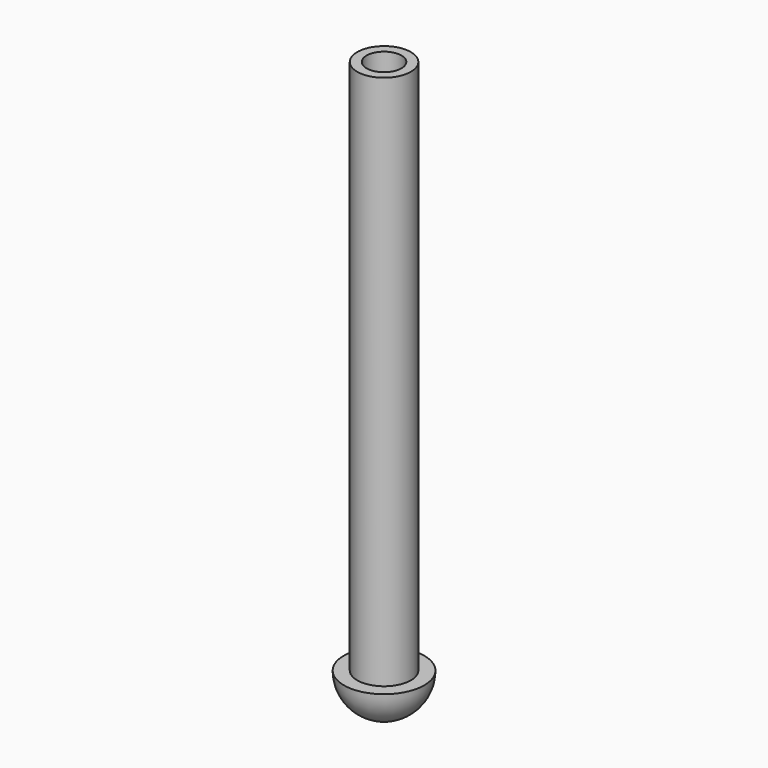
from build123d import *

# Parameters (mm, degrees)
F0_R     = 2.54
F1_DEPTH = 50.8
F3_R     = 1.651
F4_DEPTH = 6.35
F5_R     = 3.81
F6_DEPTH = 3.81
F7_R     = 3.80999


# Not quite as in the source:
# - a fillet or chamfer is up to 0.001 mm smaller than in the source, because OpenCascade refuses the exact size


with BuildPart() as f1:
    # F0 (on Top) → F1 (new body)
    with BuildSketch(Plane.XY):
        Circle(F0_R)
    extrude(amount=F1_DEPTH)

    # F3 (on face) → F4 (cut)
    with BuildSketch(Plane.XY.offset(50.8)):
        Circle(F3_R)
    extrude(amount=-F4_DEPTH, mode=Mode.SUBTRACT)

    # F5 (on face) → F6 (join)
    with BuildSketch(Plane(origin=(0, 0, 0), x_dir=(1, 0, 0), z_dir=(0, 0, -1))):
        Circle(F5_R)
    extrude(amount=F6_DEPTH)

    # F7 (radius 3.81 in the source; OpenCascade refuses exactly that, so slightly less here)
    f7_edges = [f1.edges().sort_by_distance(p)[0] for p in [
        (-3.81, 0, -3.81),
    ]]
    fillet(f7_edges, radius=F7_R)


solid = f1.part
